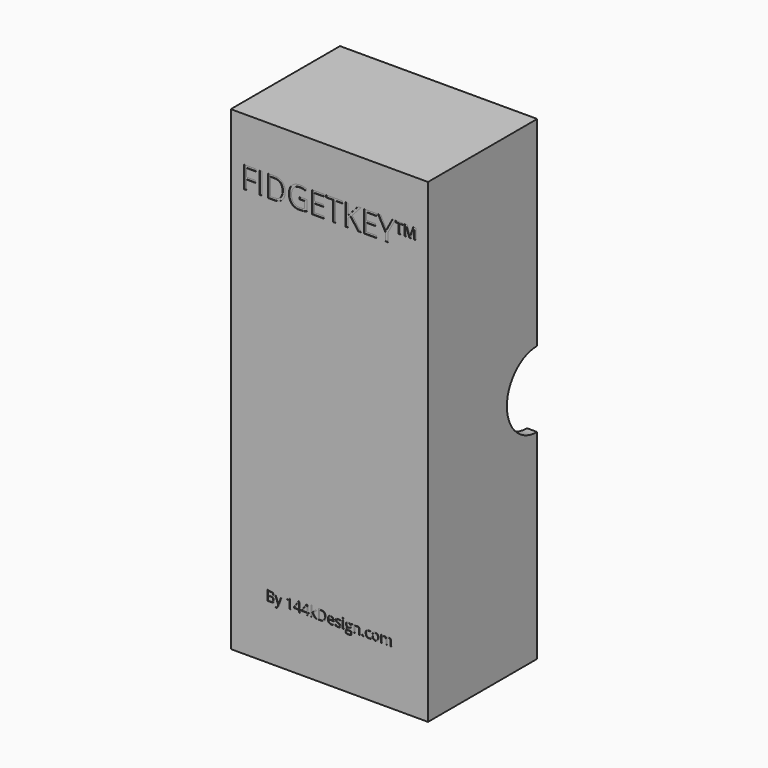
from build123d import *

# Parameters (mm, degrees)
F0_W         = 39
F0_H         = 94
F1_DEPTH     = 27
F2_T         = -2
F3_R         = 7.5
F4_DEPTH     = 25
F5_TEXT_SIZE = 5.987063666
F7_DEPTH     = 0.1
F6_TEXT_SIZE = 2.7491881304
F8_DEPTH     = 0.1


# Not quite as in the source:
# - Text() gives the source's letters only with a copy of the font that has no kerning and outlines rounded to 1/6400 em; it was checked with that copy


with BuildPart() as f1:
    # F0 (on Front) → F1 (new body)
    with BuildSketch(Plane.XZ):
        Rectangle(F0_W, F0_H)
    extrude(amount=F1_DEPTH)

    # F2
    f2_openings = [f1.faces().sort_by_distance(p)[0] for p in [
        (0, 0, 0),
    ]]
    offset(amount=F2_T, openings=f2_openings)

    # F3 (on Right) → F4 (cut, symmetric)
    with BuildSketch(Plane.YZ):
        Circle(F3_R)
    extrude(amount=F4_DEPTH, both=True, mode=Mode.SUBTRACT)

    # F5 (on face) → F7 (cut)
    with BuildSketch(Plane.XZ.offset(27)):
        with Locations((-17.5, 33.9152321065)):
            Text('FIDGETKEY™', F5_TEXT_SIZE, font='Open Sans', text_align=(TextAlign.LEFT, TextAlign.BOTTOM))
    extrude(amount=-F7_DEPTH, mode=Mode.SUBTRACT)

    # F6 (on face) → F8 (cut)
    with BuildSketch(Plane.XZ.offset(27)):
        with Locations((-12.5, -36.248188105)):
            Text('By 144kDesign.com', F6_TEXT_SIZE, font='Open Sans', text_align=(TextAlign.LEFT, TextAlign.BOTTOM))
    extrude(amount=-F8_DEPTH, mode=Mode.SUBTRACT)


solid = f1.part
